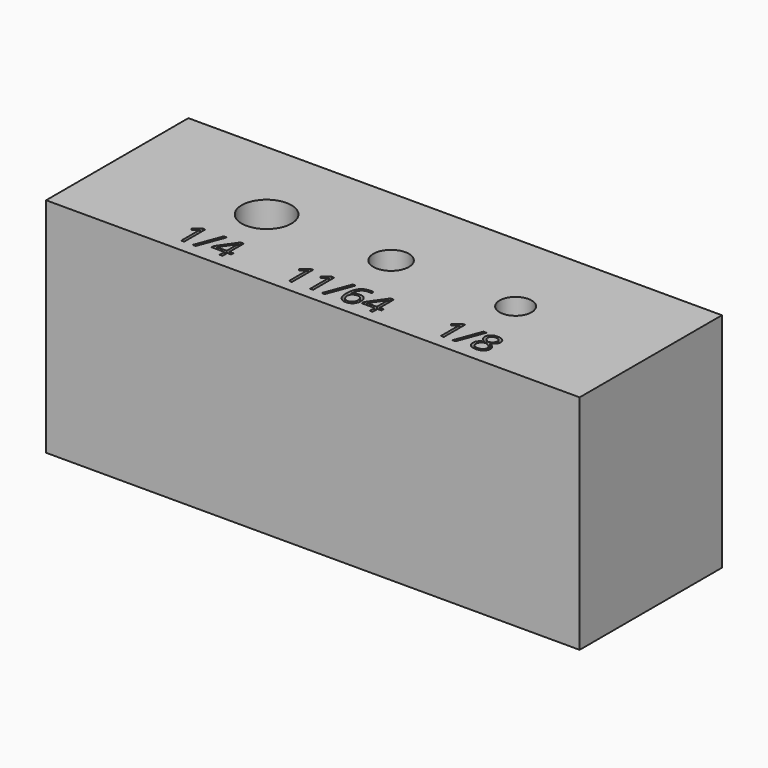
from build123d import *

# Parameters (mm, degrees)
F0_W         = 76.2
F0_H         = 25.4
F1_DEPTH     = 31.75
F3_DEPTH     = 25.4
F4_TEXT_SIZE = 5.2916666667
F5_DEPTH     = 2.54


# Not quite as in the source:
# - Text() gives the source's letters only with a copy of the font that has no kerning and outlines rounded to 1/6400 em; it was checked with that copy


with BuildPart() as f1:
    # F0 (on Top) → F1 (new body)
    with BuildSketch(Plane.XY):
        Rectangle(F0_W, F0_H)
    extrude(amount=F1_DEPTH)

    # F2 (on face) → F3 (cut)
    with BuildSketch(Plane.XY.offset(31.75)):
        with BuildLine():
            Line((-1.524, 0), (0, 0))
            Line((0, 0), (3.556, 0))
            ThreePointArc((3.556, 0), (1.016, 2.54), (-1.524, 0))
        make_face()
        with BuildLine():
            Line((3.556, 0), (0, 0))
            Line((0, 0), (-1.524, 0))
            ThreePointArc((-1.524, 0), (1.016, -2.54), (3.556, 0))
        make_face()
        with BuildLine():
            ThreePointArc((21.082, 0), (18.796, 2.286), (16.51, 0))
            Line((16.51, 0), (21.082, 0))
        make_face()
        with BuildLine():
            Line((21.082, 0), (16.51, 0))
            ThreePointArc((16.51, 0), (18.796, -2.286), (21.082, 0))
        make_face()
        with BuildLine():
            ThreePointArc((-20.32, 0), (-16.764, -3.556), (-13.208, 0))
            Line((-13.208, 0), (-20.32, 0))
        make_face()
        with BuildLine():
            Line((-20.32, 0), (-13.208, 0))
            ThreePointArc((-13.208, 0), (-16.764, 3.556), (-20.32, 0))
        make_face()
    extrude(amount=-F3_DEPTH, mode=Mode.SUBTRACT)

    # F4 (on face) → F5 (cut)
    with BuildSketch(Plane.XY.offset(31.75)):
        with Locations((-21.6720713027, -10.9037882781)):
            Text('1/4', F4_TEXT_SIZE, font='Open Sans', text_align=(TextAlign.LEFT, TextAlign.BOTTOM))
        with Locations((-6.2027975276, -10.9968022443)):
            Text('11/64', F4_TEXT_SIZE, font='Open Sans', text_align=(TextAlign.LEFT, TextAlign.BOTTOM))
        with Locations((15.322955339, -10.7811833732)):
            Text('1/8', F4_TEXT_SIZE, font='Open Sans', text_align=(TextAlign.LEFT, TextAlign.BOTTOM))
    extrude(amount=-F5_DEPTH, mode=Mode.SUBTRACT)


solid = f1.part
